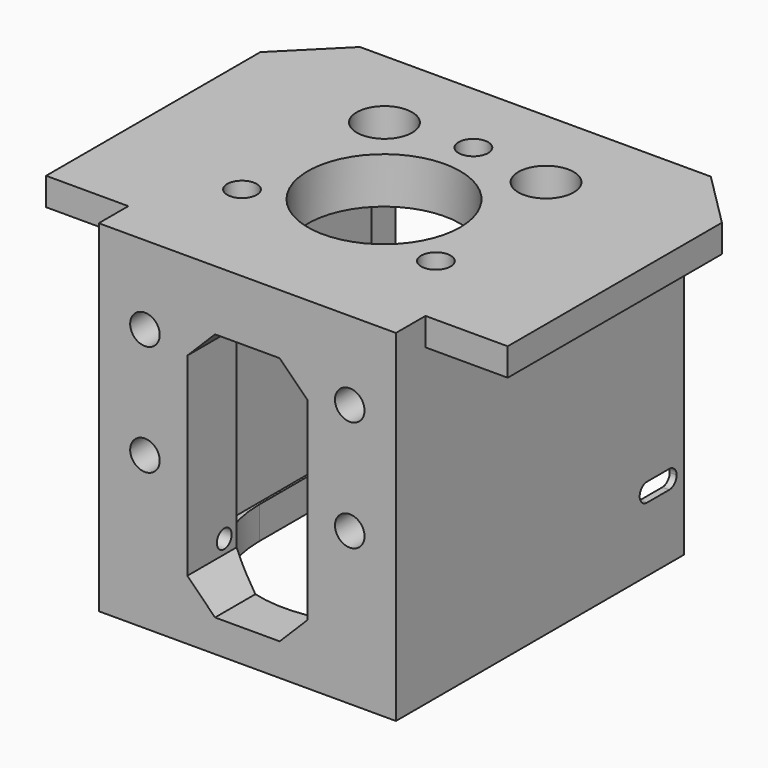
from build123d import *
from build123d import SkipClean  # not in build123d's __all__

# Parameters (mm, degrees)
F0_R      = 1.6
F0_R_2    = 8.25
F0_R_3    = 3
F1_DEPTH  = 3
F2_R      = 3
F2_R_2    = 1.6
F2_R_3    = 8.25
F3_DEPTH  = 34
F4_W      = 30.5
F4_H      = 30.5
F5_DEPTH  = 5
F6_W      = 27.5
F6_H      = 28.5
F7_DEPTH  = 24.77
F9_DEPTH  = 32
F10_R     = 1.6
F11_DEPTH = 39.001
F12_R     = 1.6
F13_DEPTH = 2
F15_DEPTH = 4
F16_R     = 1.6
F17_DEPTH = 4
F20_R     = 1.2
F21_DEPTH = 5
F22_R     = 1
F23_DEPTH = 9.591955051
F25_DEPTH = 2.342955051


# Not quite as in the source:
# - after a boolean that leaves OpenCascade's solid faulty, fix() repairs it


with BuildPart() as f1:
    # F0 (on Top) → F1 (new body)
    with BuildSketch(Plane.XY):
        Polygon((-25, 29), (-25, 0), (-16.091955051, 0), (-16.091955051, -4), (16.091955051, -4), (16.091955051, 0), (25, 0), (25, 29), (19, 35), (-19, 35), align=None)
        with Locations((-10.5, 8.4)):
            Circle(F0_R, mode=Mode.SUBTRACT)
        with Locations((10.5, 8.4)):
            Circle(F0_R, mode=Mode.SUBTRACT)
        with Locations((0, 14.5)):
            Circle(F0_R_2, mode=Mode.SUBTRACT)
        with Locations((-8.75, 25.5)):
            Circle(F0_R_3, mode=Mode.SUBTRACT)
        with Locations((0, 26.6)):
            Circle(F0_R, mode=Mode.SUBTRACT)
        with Locations((8.75, 25.5)):
            Circle(F0_R_3, mode=Mode.SUBTRACT)
    extrude(amount=F1_DEPTH)

    # F2 (on face) → F3 (join)
    with BuildSketch(Plane(origin=(0, 0, 0), x_dir=(1, 0, 0), z_dir=(0, 0, -1))):
        Polygon((16.091955051, 4), (-16.091955051, 4), (-16.091955051, 0), (-16.091955051, -35), (16.091955051, -35), (16.091955051, 0), align=None)
        with Locations((-8.75, -25.5)):
            Circle(F2_R, mode=Mode.SUBTRACT)
        with Locations((0, -26.6)):
            Circle(F2_R_2, mode=Mode.SUBTRACT)
        with Locations((8.75, -25.5)):
            Circle(F2_R, mode=Mode.SUBTRACT)
        with Locations((-10.5, -8.4)):
            Circle(F2_R_2, mode=Mode.SUBTRACT)
        with Locations((0, -14.5)):
            Circle(F2_R_3, mode=Mode.SUBTRACT)
        with Locations((10.5, -8.4)):
            Circle(F2_R_2, mode=Mode.SUBTRACT)
    extrude(amount=F3_DEPTH)

    # F4 (on face) → F5 (cut)
    with BuildSketch(Plane(origin=(0, 35, 0), x_dir=(-1, 0, 0), z_dir=(0, 1, 0))):
        with Locations((-0.091955051, -15.25)):
            Rectangle(F4_W, F4_H)
    extrude(amount=-F5_DEPTH, mode=Mode.SUBTRACT)

    # F6 (on face) → F7 (cut)
    with BuildSketch(Plane(origin=(0, 30, 0), x_dir=(-1, 0, 0), z_dir=(0, 1, 0))):
        with Locations((0, -16.25)):
            Rectangle(F6_W, F6_H)
    extrude(amount=-F7_DEPTH, mode=Mode.SUBTRACT)

    # F8 (on face) → F9 (cut)
    with BuildSketch(Plane(origin=(0, 0, -34), x_dir=(1, 0, 0), z_dir=(0, 0, -1))):
        with BuildLine():
            Line((8.25, -14.5), (13.5, -14.5))
            ThreePointArc((13.5, -14.5), (13.1444351182, -11.4220420042), (12.0964703076, -8.5062193819))
            ThreePointArc((12.0964703076, -8.5062193819), (9.1165222882, -9.2037346707), (11.1984910379, -6.9605173603))
            ThreePointArc((11.1984910379, -6.9605173603), (0, -1), (-11.1984910379, -6.9605173603))
            ThreePointArc((-11.1984910379, -6.9605173603), (-9.6507608289, -7.043979045), (-8.9, -8.4))
            ThreePointArc((-8.9, -8.4), (-10.4468609941, -9.9991173334), (-12.0964703076, -8.5062193819))
            ThreePointArc((-12.0964703076, -8.5062193819), (-13.1444351182, -11.4220420042), (-13.5, -14.5))
            Line((-13.5, -14.5), (-8.25, -14.5))
            ThreePointArc((-8.25, -14.5), (0, -6.25), (8.25, -14.5))
        make_face()
        with BuildLine():
            Line((13.5, -35), (13.5, -14.5))
            ThreePointArc((13.5, -14.5), (12.717238531, -19.0301042091), (10.4597267933, -23.0348764144))
            ThreePointArc((10.4597267933, -23.0348764144), (11.4079296812, -24.1088099303), (11.75, -25.5))
            ThreePointArc((11.75, -25.5), (9.3158770477, -28.4461471733), (5.9634778888, -26.611438043))
            ThreePointArc((5.9634778888, -26.611438043), (3.4585284768, -27.5494666855), (0.8178060745, -27.9752066116))
            ThreePointArc((0.8178060745, -27.9752066116), (0, -28.2), (-0.8178060745, -27.9752066116))
            ThreePointArc((-0.8178060745, -27.9752066116), (-3.4585284768, -27.5494666855), (-5.9634778888, -26.611438043))
            ThreePointArc((-5.9634778888, -26.611438043), (-10.6175706975, -27.8478031625), (-10.4597267933, -23.0348764144))
            ThreePointArc((-10.4597267933, -23.0348764144), (-12.717238531, -19.0301042091), (-13.5, -14.5))
            Line((-13.5, -14.5), (-13.5, -35))
            Line((-13.5, -35), (13.5, -35))
        make_face()
        with BuildLine():
            ThreePointArc((10.4597267933, -23.0348764144), (12.717238531, -19.0301042091), (13.5, -14.5))
            Line((13.5, -14.5), (8.25, -14.5))
            ThreePointArc((8.25, -14.5), (0, -22.75), (-8.25, -14.5))
            Line((-8.25, -14.5), (-13.5, -14.5))
            ThreePointArc((-13.5, -14.5), (-12.717238531, -19.0301042091), (-10.4597267933, -23.0348764144))
            ThreePointArc((-10.4597267933, -23.0348764144), (-7.3588099303, -22.8420703188), (-5.75, -25.5))
            ThreePointArc((-5.75, -25.5), (-5.8038528267, -26.0658770477), (-5.9634778888, -26.611438043))
            ThreePointArc((-5.9634778888, -26.611438043), (-3.4585284768, -27.5494666855), (-0.8178060745, -27.9752066116))
            ThreePointArc((-0.8178060745, -27.9752066116), (-0.7910468636, -25.2092286818), (1.6, -26.6))
            ThreePointArc((1.6, -26.6), (1.3907713182, -27.3910468636), (0.8178060745, -27.9752066116))
            ThreePointArc((0.8178060745, -27.9752066116), (3.4585284768, -27.5494666855), (5.9634778888, -26.611438043))
            ThreePointArc((5.9634778888, -26.611438043), (6.8824293025, -23.1521968375), (10.4597267933, -23.0348764144))
        make_face()
        with BuildLine():
            ThreePointArc((11.1984910379, -6.9605173603), (9.1165222882, -9.2037346707), (12.0964703076, -8.5062193819))
            ThreePointArc((12.0964703076, -8.5062193819), (11.6730931936, -7.7184887161), (11.1984910379, -6.9605173603))
        make_face()
    extrude(amount=-F9_DEPTH, mode=Mode.SUBTRACT)

    # F10 (on face) → F11 (cut, through all)
    with BuildSketch(Plane.XZ.offset(4)):
        with Locations((-11.091955051, -5.5)):
            Circle(F10_R)
        Polygon((-3.5, -3.5), (-6.5, -6.5), (-6.5, -27.5), (-3.5, -30.5), (3.5, -30.5), (6.5, -27.5), (6.5, -6.5), (3.5, -3.5), align=None)
        with Locations((-11.091955051, -17.5)):
            Circle(F10_R)
        with Locations((11.091955051, -17.5)):
            Circle(F10_R)
        with Locations((11.091955051, -5.5)):
            Circle(F10_R)
    extrude(amount=-F11_DEPTH, mode=Mode.SUBTRACT)

    # F12 (on face) → F13 (cut)
    with BuildSketch(Plane(origin=(0, 0, -2), x_dir=(1, 0, 0), z_dir=(0, 0, -1))):
        Polygon((-8.8689854895, -11.225), (-7.2379709791, -8.4), (-8.8689854895, -5.575), (-12.1310145105, -5.575), (-13.75, -8.3791651246), (-13.75, -8.4208348754), (-12.1310145105, -11.225), align=None)
        with Locations((-10.5, -8.4)):
            Circle(F12_R, mode=Mode.SUBTRACT)
        Polygon((12.1310145105, -11.225), (13.75, -8.4208348754), (13.75, -8.3791651246), (12.1310145105, -5.575), (8.8689854895, -5.575), (7.2379709791, -8.4), (8.8689854895, -11.225), align=None)
        with Locations((10.5, -8.4)):
            Circle(F12_R, mode=Mode.SUBTRACT)
        Polygon((1.6310145105, -29.425), (3.2620290209, -26.6), (1.6310145105, -23.775), (-1.6310145105, -23.775), (-3.2620290209, -26.6), (-1.6310145105, -29.425), align=None)
        with Locations((0, -26.6)):
            Circle(F12_R, mode=Mode.SUBTRACT)
    extrude(amount=-F13_DEPTH, mode=Mode.SUBTRACT)

    # F14 (on face) → F15 (join)
    with BuildSketch(Plane(origin=(0, 0, -2), x_dir=(1, 0, 0), z_dir=(0, 0, -1))):
        with BuildLine():
            Line((-13.75, -30), (-9.25, -30))
            Line((-9.25, -30), (-9.25, -28.4580398915))
            ThreePointArc((-9.25, -28.4580398915), (-11.1952034569, -27.2380966757), (-11.7080398915, -25))
            Line((-11.7080398915, -25), (-13.75, -25))
            Line((-13.75, -25), (-13.75, -30))
        make_face()
        with BuildLine():
            Line((9.25, -30), (13.75, -30))
            Line((13.75, -30), (13.75, -25))
            Line((13.75, -25), (11.7080398915, -25))
            ThreePointArc((11.7080398915, -25), (11.7394915684, -25.2491212192), (11.75, -25.5))
            ThreePointArc((11.75, -25.5), (11.0412878475, -27.4364916731), (9.25, -28.4580398915))
            Line((9.25, -28.4580398915), (9.25, -30))
        make_face()
    with SkipClean():  # cleaning this boolean's faces spoils the solid; the shape is the same uncleaned
        extrude(amount=F15_DEPTH)


with BuildPart() as f17:
    # F16 (on face) → F17 (new body)
    with BuildSketch(Plane.XZ.offset(4)):
        Polygon((-11.091955051, -8.7620290209), (-8.266955051, -7.1310145105), (-8.266955051, -3.8689854895), (-11.091955051, -2.2379709791), (-13.916955051, -3.8689854895), (-13.916955051, -7.1310145105), align=None)
        with Locations((-11.091955051, -5.5)):
            Circle(F16_R, mode=Mode.SUBTRACT)
    extrude(amount=F17_DEPTH)


with BuildPart() as f17b:
    # F16 (on face) → F17, piece 2 (new body)
    with BuildSketch(Plane.XZ.offset(4)):
        Polygon((-11.091955051, -20.7620290209), (-8.266955051, -19.1310145105), (-8.266955051, -15.8689854895), (-11.091955051, -14.2379709791), (-13.916955051, -15.8689854895), (-13.916955051, -19.1310145105), align=None)
        with Locations((-11.091955051, -17.5)):
            Circle(F16_R, mode=Mode.SUBTRACT)
    extrude(amount=F17_DEPTH)


with BuildPart() as f17c:
    # F16 (on face) → F17, piece 3 (new body)
    with BuildSketch(Plane.XZ.offset(4)):
        Polygon((11.091955051, -20.7620290209), (13.916955051, -19.1310145105), (13.916955051, -15.8689854895), (11.091955051, -14.2379709791), (8.266955051, -15.8689854895), (8.266955051, -19.1310145105), align=None)
        with Locations((11.091955051, -17.5)):
            Circle(F16_R, mode=Mode.SUBTRACT)
    extrude(amount=F17_DEPTH)


with BuildPart() as f17d:
    # F16 (on face) → F17, piece 4 (new body)
    with BuildSketch(Plane.XZ.offset(4)):
        Polygon((11.091955051, -8.7620290209), (13.916955051, -7.1310145105), (13.916955051, -3.8689854895), (11.091955051, -2.2379709791), (8.266955051, -3.8689854895), (8.266955051, -7.1310145105), align=None)
        with Locations((11.091955051, -5.5)):
            Circle(F16_R, mode=Mode.SUBTRACT)
    extrude(amount=F17_DEPTH)


with BuildPart() as f17_1:
    # F18: moved
    add(f17.part.moved(Location((0, 10.3, 0))), clean=False)


with BuildPart() as f17b_1:
    # F18: moved
    add(f17b.part.moved(Location((0, 10.3, 0))), clean=False)


with BuildPart() as f17d_1:
    # F18: moved
    add(f17d.part.moved(Location((0, 10.3, 0))), clean=False)


with BuildPart() as f17c_1:
    # F18: moved
    add(f17c.part.moved(Location((0, 10.3, 0))), clean=False)


with BuildPart() as f1_1:
    add(f1.part, clean=False)

    # F19: cut F17, F17b, F17d, F17c
    add(f17_1.part, mode=Mode.SUBTRACT)
    add(f17b_1.part, mode=Mode.SUBTRACT)
    add(f17d_1.part, mode=Mode.SUBTRACT)
    add(f17c_1.part, mode=Mode.SUBTRACT)

    add(f1_1.part.fix(), mode=Mode.REPLACE)

    # F20 (on face) → F21 (cut, through all)
    with BuildSketch(Plane(origin=(0, 30, 0), x_dir=(-1, 0, 0), z_dir=(0, 1, 0))):
        with Locations((-12, -3.25)):
            Circle(F20_R)
        with Locations((12, -3.25)):
            Circle(F20_R)
    extrude(amount=-F21_DEPTH, mode=Mode.SUBTRACT)

    # F22 (on face) → F23 (cut, through all)
    with BuildSketch(Plane(origin=(-16.091955051, 0, 0), x_dir=(0, -1, 0), z_dir=(-1, 0, 0))):
        with Locations((-1, -26)):
            Circle(F22_R)
    extrude(amount=-F23_DEPTH, mode=Mode.SUBTRACT)

    # F24 (on face) → F25 (cut, through all)
    with BuildSketch(Plane.YZ.offset(16.091955051)):
        with BuildLine():
            ThreePointArc((30, -27), (30.7071067812, -26.7071067812), (31, -26))
            ThreePointArc((31, -26), (30.7071067812, -25.2928932188), (30, -25))
            Line((30, -25), (30, -27))
        make_face()
        with BuildLine():
            Line((30, -27), (30, -25))
            ThreePointArc((30, -25), (29, -26), (30, -27))
        make_face()
        with BuildLine():
            ThreePointArc((30, -25), (30.7071067812, -25.2928932188), (31, -26))
            ThreePointArc((31, -26), (30.7071067812, -26.7071067812), (30, -27))
            Line((30, -27), (33, -27))
            ThreePointArc((33, -27), (32, -26), (33, -25))
            Line((33, -25), (30, -25))
        make_face()
        with BuildLine():
            ThreePointArc((34, -26), (33.7071067812, -25.2928932188), (33, -25))
            Line((33, -25), (33, -27))
            ThreePointArc((33, -27), (33.7071067812, -26.7071067812), (34, -26))
        make_face()
        with BuildLine():
            Line((33, -27), (33, -25))
            ThreePointArc((33, -25), (32, -26), (33, -27))
        make_face()
    extrude(amount=-F25_DEPTH, mode=Mode.SUBTRACT)


solid = f1_1.part
